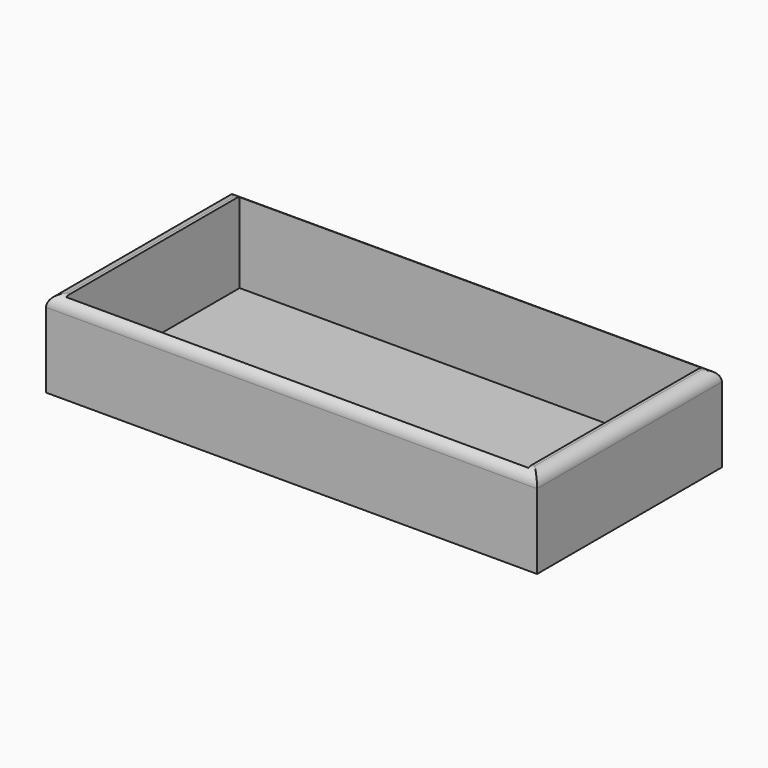
from build123d import *

# Parameters (mm, degrees)
F0_W        = 170
F0_H        = 80
F1_DEPTH    = 30
F2_W        = 160
F2_H        = 75
F3_DEPTH    = 28
F4_T1_DEPTH = 190
F4_T3_DEPTH = 100


# Not quite as in the source:
# - a fillet or chamfer that OpenCascade refuses, or shapes differently, is made with other operations: its cross-section is extruded or revolved along the edge and cut away or added


with BuildPart() as f1:
    # F0 (on Top) → F1 (new body)
    with BuildSketch(Plane.XY):
        Rectangle(F0_W, F0_H)
    extrude(amount=F1_DEPTH)

    # F2 (on face) → F3 (cut)
    with BuildSketch(Plane.XY.offset(30)):
        Rectangle(F2_W, F2_H)
    extrude(amount=-F3_DEPTH, mode=Mode.SUBTRACT)

    # F4: fillet of radius 4 on 4 edges, made by hand

    # F4_s2 → F4_t1 (cut)
    with BuildSketch(Plane.YZ.offset(-95)):
        with BuildLine():
            ThreePointArc((-40, 26), (-38.8284271247, 28.8284271247), (-36, 30))
            Line((-36, 30), (-40, 30))
            Line((-40, 30), (-40, 26))
        make_face()
        with BuildLine():
            ThreePointArc((40, 26), (38.8284271247, 28.8284271247), (36, 30))
            Line((36, 30), (40, 30))
            Line((40, 30), (40, 26))
        make_face()
    extrude(amount=F4_T1_DEPTH, mode=Mode.SUBTRACT)

    # F4_s4 → F4_t3 (cut)
    with BuildSketch(Plane.XZ.offset(-50)):
        with BuildLine():
            ThreePointArc((-85, 26), (-83.8284271247, 28.8284271247), (-81, 30))
            Line((-81, 30), (-85, 30))
            Line((-85, 30), (-85, 26))
        make_face()
        with BuildLine():
            ThreePointArc((81, 30), (83.8284271247, 28.8284271247), (85, 26))
            Line((85, 26), (85, 30))
            Line((85, 30), (81, 30))
        make_face()
    extrude(amount=F4_T3_DEPTH, mode=Mode.SUBTRACT)


solid = f1.part
